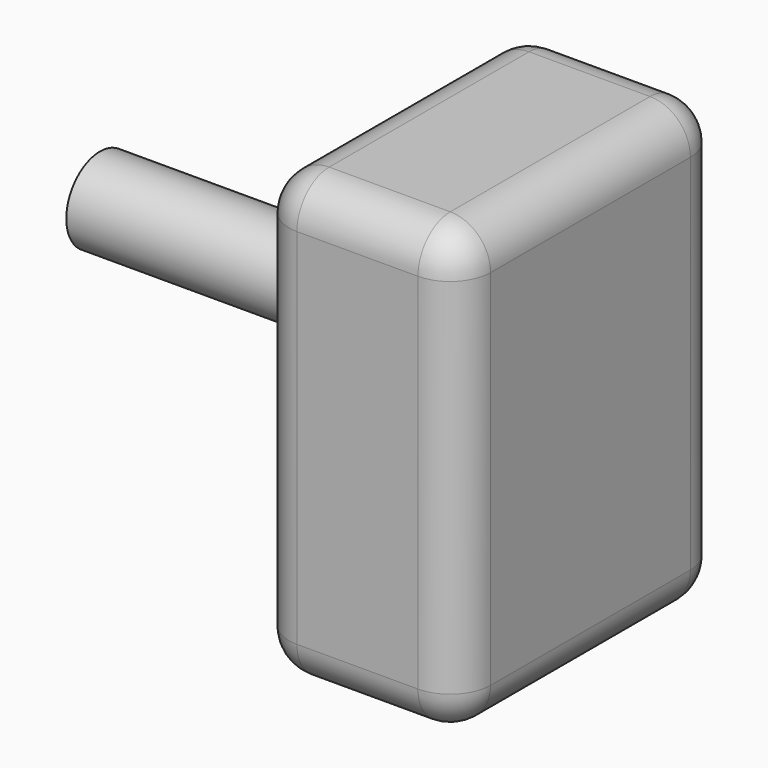
from build123d import *

# Parameters (mm, degrees)
F2_W         = 41.6020527482
F2_H         = 55.9058710933
F3_DEPTH     = 25.4
F4_R         = 5.08
F5_T1_DEPTH  = 45.7458710933
F5_T3_DEPTH  = 31.4420527482
F5_T5_DEPTH  = 15.24
F5_S9_W      = 5.08
F5_S9_H      = 5.08
F5_T10_DEPTH = 5.08
F5_S15_W     = 5.08
F5_S15_H     = 5.08
F5_T16_DEPTH = 5.08
F5_S21_W     = 5.08
F5_S21_H     = 5.08
F5_T22_DEPTH = 5.08
F5_S27_W     = 5.08
F5_S27_H     = 5.08
F5_T28_DEPTH = 5.08
F7_DEPTH     = 25.4
F8_R         = 5.2966255489
F9_DEPTH     = 67.6975995302


# Not quite as in the source:
# - a fillet or chamfer that OpenCascade refuses, or shapes differently, is made with other operations: its cross-section is extruded or revolved along the edge and cut away or added


with BuildPart() as f3:
    # F2 (on face) → F3 (new body)
    with BuildSketch(Plane.YZ):
        with Locations((20.8010263741, 27.9529355466)):
            Rectangle(F2_W, F2_H)
    extrude(amount=F3_DEPTH)

    # F4
    f4_edges = [f3.edges().sort_by_distance(p)[0] for p in [
        (12.7, 0, 0),
        (12.7, 41.602053, 0),
        (0, 20.801026, 0),
        (25.4, 20.801026, 0),
        (25.4, 41.602053, 27.952936),
        (25.4, 20.801026, 55.905871),
        (25.4, 0, 27.952936),
        (12.7, 41.602053, 55.905871),
        (0, 41.602053, 27.952936),
    ]]
    fillet(f4_edges, radius=F4_R)

    # F5: fillet of radius 5.08 on 3 edges, made by hand

    # F5_s2 → F5_t1 (cut)
    with BuildSketch(Plane.XY.offset(5.08)):
        with BuildLine():
            ThreePointArc((0, 5.08), (1.4878975516, 1.4878975516), (5.08, 0))
            Line((5.08, 0), (0, 0))
            Line((0, 0), (0, 5.08))
        make_face()
    extrude(amount=F5_T1_DEPTH, mode=Mode.SUBTRACT)

    # F5_s4 → F5_t3 (cut)
    with BuildSketch(Plane.XZ.offset(-36.5220527482)):
        with BuildLine():
            ThreePointArc((0, 50.8258710933), (1.4878975516, 54.4179735417), (5.08, 55.9058710933))
            Line((5.08, 55.9058710933), (0, 55.9058710933))
            Line((0, 55.9058710933), (0, 50.8258710933))
        make_face()
    extrude(amount=F5_T3_DEPTH, mode=Mode.SUBTRACT)

    # F5_s6 → F5_t5 (cut)
    with BuildSketch(Plane.YZ.offset(5.08)):
        with BuildLine():
            ThreePointArc((5.08, 55.9058710933), (1.4878975516, 54.4179735417), (0, 50.8258710933))
            Line((0, 50.8258710933), (0, 55.9058710933))
            Line((0, 55.9058710933), (5.08, 55.9058710933))
        make_face()
    extrude(amount=F5_T5_DEPTH, mode=Mode.SUBTRACT)


with BuildPart() as f5_tool8:
    # F5_s9 → F5_t10 (new body)
    with BuildSketch(Plane.XY.offset(50.8258710933)):
        with Locations((22.86, 2.54)):
            Rectangle(F5_S9_W, F5_S9_H)
    extrude(amount=F5_T10_DEPTH)

    # F5_s11 → F5_t12 (revolve, cut)
    with BuildSketch(Plane(origin=(20.32, 5.08, 50.8258710933), x_dir=(-0.7071067812, 0.7071067812, 0), z_dir=(0.7071067812, 0.7071067812, 0))):
        with BuildLine():
            ThreePointArc((0, -5.08), (5.08, 0), (0, 5.08))
            Line((0, 5.08), (0, -5.08))
        make_face()
    revolve(axis=Axis((20.32, 5.08, 50.8258710933), (0, 0, 1)), mode=Mode.SUBTRACT)


with BuildPart() as f3_1:
    add(f3.part)

    # F5_t7: cut F5_tool8
    add(f5_tool8.part, mode=Mode.SUBTRACT)


with BuildPart() as f5_tool14:
    # F5_s15 → F5_t16 (new body)
    with BuildSketch(Plane.YZ.offset(5.08)):
        with Locations((39.0620527482, 53.3658710933)):
            Rectangle(F5_S15_W, F5_S15_H)
    extrude(amount=-F5_T16_DEPTH)

    # F5_s17 → F5_t18 (revolve, cut)
    with BuildSketch(Plane(origin=(5.08, 36.5220527482, 50.8258710933), x_dir=(0, -0.7071067812, -0.7071067812), z_dir=(0, 0.7071067812, -0.7071067812))):
        with BuildLine():
            ThreePointArc((0, -5.08), (5.08, 0), (0, 5.08))
            Line((0, 5.08), (0, -5.08))
        make_face()
    revolve(axis=Axis((5.08, 36.5220527482, 50.8258710933), (-1, 0, 0)), mode=Mode.SUBTRACT)


with BuildPart() as f3_2:
    add(f3_1.part)

    # F5_t13: cut F5_tool14
    add(f5_tool14.part, mode=Mode.SUBTRACT)


with BuildPart() as f5_tool20:
    # F5_s21 → F5_t22 (new body)
    with BuildSketch(Plane.YZ.offset(5.08)):
        with Locations((2.54, 2.54)):
            Rectangle(F5_S21_W, F5_S21_H)
    extrude(amount=-F5_T22_DEPTH)

    # F5_s23 → F5_t24 (revolve, cut)
    with BuildSketch(Plane(origin=(5.08, 5.08, 5.08), x_dir=(0, 0.7071067812, 0.7071067812), z_dir=(0, -0.7071067812, 0.7071067812))):
        with BuildLine():
            ThreePointArc((0, -5.08), (5.08, 0), (0, 5.08))
            Line((0, 5.08), (0, -5.08))
        make_face()
    revolve(axis=Axis((5.08, 5.08, 5.08), (-1, 0, 0)), mode=Mode.SUBTRACT)


with BuildPart() as f3_3:
    add(f3_2.part)

    # F5_t19: cut F5_tool20
    add(f5_tool20.part, mode=Mode.SUBTRACT)


with BuildPart() as f5_tool26:
    # F5_s27 → F5_t28 (new body)
    with BuildSketch(Plane.YZ.offset(5.08)):
        with Locations((2.54, 53.3658710933)):
            Rectangle(F5_S27_W, F5_S27_H)
    extrude(amount=-F5_T28_DEPTH)

    # F5_s29 → F5_t30 (revolve, cut)
    with BuildSketch(Plane(origin=(5.08, 5.08, 50.8258710933), x_dir=(0, 0.7071067812, -0.7071067812), z_dir=(0, 0.7071067812, 0.7071067812))):
        with BuildLine():
            ThreePointArc((0, -5.08), (5.08, 0), (0, 5.08))
            Line((0, 5.08), (0, -5.08))
        make_face()
    revolve(axis=Axis((5.08, 5.08, 50.8258710933), (-1, 0, 0)), mode=Mode.SUBTRACT)


with BuildPart() as f3_4:
    add(f3_3.part)

    # F5_t25: cut F5_tool26
    add(f5_tool26.part, mode=Mode.SUBTRACT)

    # F6 (on face) → F7 (cut)
    with BuildSketch(Plane.YZ.offset(25.4)):
        with BuildLine():
            ThreePointArc((28.6198008208, 24.1723779255), (30.5921769571, 25.8541960079), (31.3290304018, 28.3393170685))
            ThreePointArc((31.3290304018, 28.3393170685), (28.3928704941, 32.5997711108), (23.3662914361, 31.3725764954))
            ThreePointArc((23.3662914361, 31.3725764954), (26.7699286342, 28.3393170685), (28.6198008208, 24.1723779255))
        make_face()
        with BuildLine():
            ThreePointArc((28.6198008208, 24.1723779255), (26.7699286342, 28.3393170685), (23.3662914361, 31.3725764954))
            ThreePointArc((23.3662914361, 31.3725764954), (23.0869595481, 25.652097755), (28.6198008208, 24.1723779255))
        make_face()
        with BuildLine():
            ThreePointArc((28.6198008208, 24.1723779255), (23.0869595481, 25.652097755), (23.3662914361, 31.3725764954))
            ThreePointArc((23.3662914361, 31.3725764954), (8.7034109088, 16.5279412286), (28.8466709714, 21.9696629792))
            ThreePointArc((28.8466709714, 21.9696629792), (28.7898038098, 23.0768467038), (28.6198008208, 24.1723779255))
        make_face()
    extrude(amount=F7_DEPTH, mode=Mode.SUBTRACT)

    # F8 (on face) → F9 (join)
    with BuildSketch(Plane.YZ.offset(25.4)):
        with Locations((28.2216444612, 27.5326687843)):
            Circle(F8_R)
    extrude(amount=-F9_DEPTH)


solid = f3_4.part
